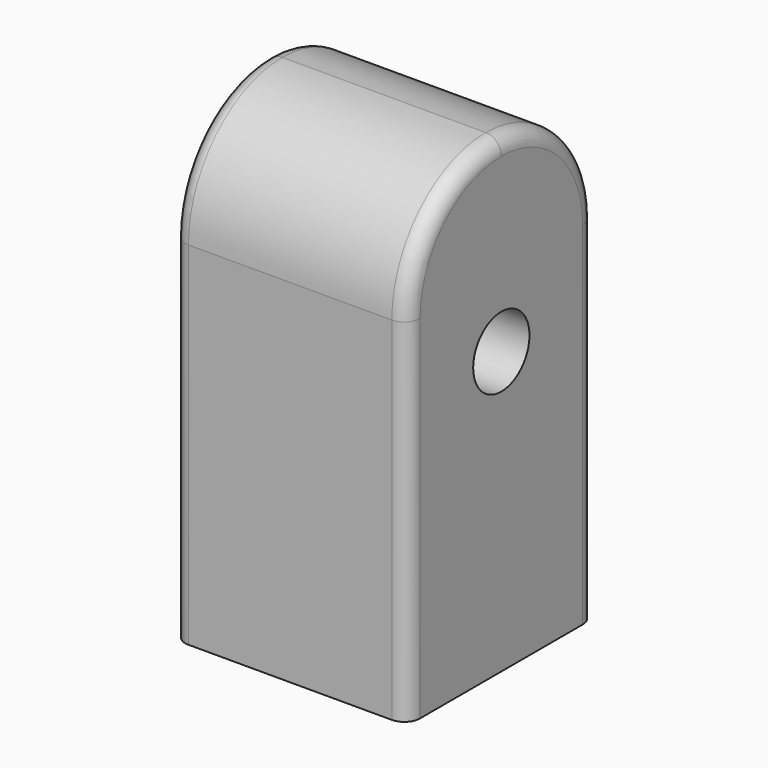
from build123d import *

# Parameters (mm, degrees)
F0_W     = 30
F0_H     = 60
F1_DEPTH = 15
F3_R     = 14.99999
F4_R     = 2
F5_D     = 9


# Not quite as in the source:
# - a fillet or chamfer is up to 0.001 mm smaller than in the source, because OpenCascade refuses the exact size


with BuildPart() as f1:
    # F0 (on Right) → F1 (new body, symmetric)
    with BuildSketch(Plane.YZ):
        Rectangle(F0_W, F0_H)
    extrude(amount=F1_DEPTH, both=True)

    # F3 (radius 15 in the source; OpenCascade refuses exactly that, so slightly less here)
    f3_edges = [f1.edges().sort_by_distance(p)[0] for p in [
        (0, -15, 30),
        (0, 15, 30),
    ]]
    fillet(f3_edges, radius=F3_R)

    # F4
    f4_edges = [f1.edges().sort_by_distance(p)[0] for p in [
        (15, -15, -7.499995),
        (-15, 15, -7.499995),
        (-15, -10.606605, 25.606605),
    ]]
    fillet(f4_edges, radius=F4_R)

    # F5 (through all)
    with Locations(Plane.YZ.offset(15)):
        with Locations((0, 6)):
            Hole(F5_D / 2)


solid = f1.part
